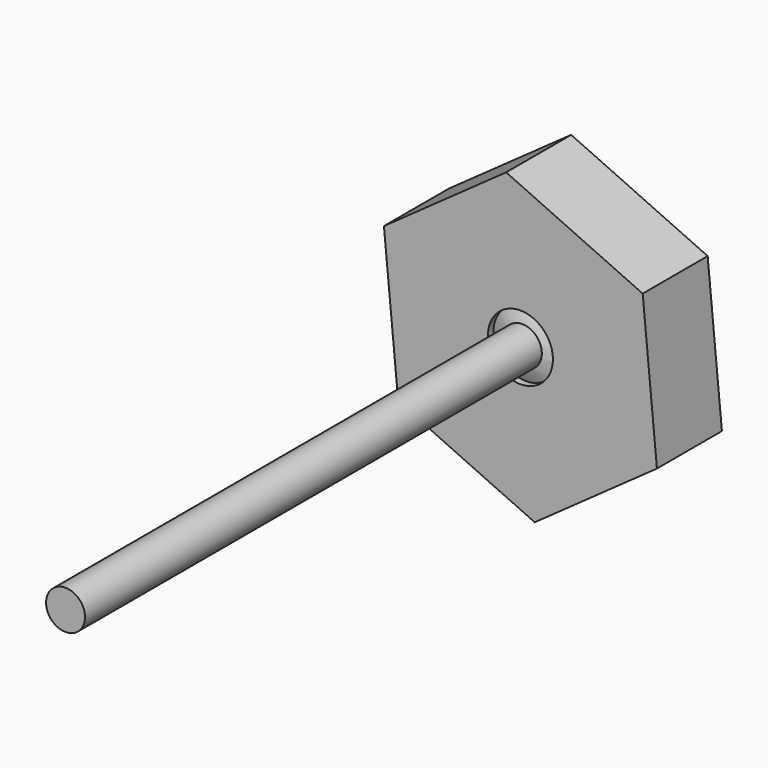
from build123d import *

# Parameters (mm, degrees)
F2_R     = 6
F3_DEPTH = 200
F4_R     = 10
F5_DEPTH = 25


with BuildPart() as f1:
    # F0 (on Front) → F1 (revolve)
    with BuildSketch(Plane.XZ):
        with BuildLine():
            Line((0, 25), (0, -25))
            ThreePointArc((0, -25), (25, 0), (0, 25))
        make_face()
    revolve(axis=Axis((0, 0, 0), (0, 0, 1)))

    # F2 (on Front) → F3 (join)
    with BuildSketch(Plane.XZ):
        Circle(F2_R)
    extrude(amount=F3_DEPTH)


with BuildPart() as f5:
    # F4 (on Front) → F5 (new body)
    with BuildSketch(Plane.XZ):
        Polygon((-42.0127453861, 19.1901682759), (-37.6255459229, -26.7890206491), (4.3871994632, -45.979188925), (42.0127453861, -19.1901682759), (37.6255459229, 26.7890206491), (-4.3871994632, 45.979188925), align=None)
        Circle(F4_R, mode=Mode.SUBTRACT)
    extrude(amount=F5_DEPTH)

    # F6 (on Right) → F7 (revolve, cut)
    with BuildSketch(Plane.YZ):
        with BuildLine():
            Line((0, 25), (0, -25))
            ThreePointArc((0, -25), (25, 0), (0, 25))
        make_face()
    revolve(axis=Axis((0, 0, 0), (0, 0, 1)), mode=Mode.SUBTRACT)


solid = Compound([f1.part, f5.part])
